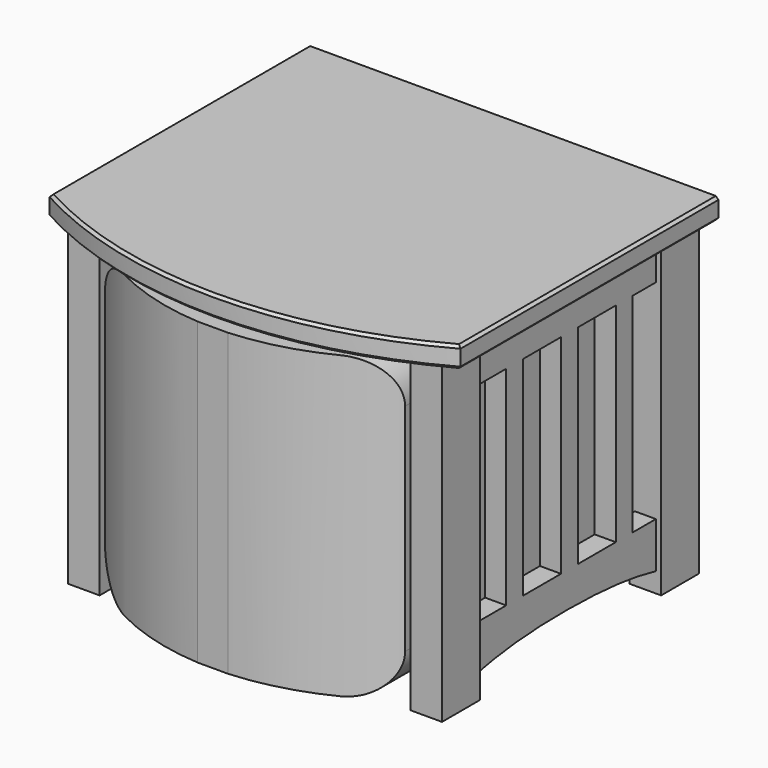
from build123d import *

# Parameters (mm, degrees)
F4_DEPTH  = 425.45
F5_R      = 19.05
F6_DEPTH  = 9.525
F8_DEPTH  = 361.95
F9_W      = 57.15
F9_H      = 381.0128062427
F10_DEPTH = 38.1
F9_H_2    = 381
F11_W     = 57.15
F11_H     = 251.1923307657
F12_DEPTH = 25.4
F16_DEPTH = 25.4
F17_SIZE  = 3.175
F18_W     = 374.65
F18_H     = 25.4
F19_DEPTH = 19.05


# Not quite as in the source:
# - a feature names something its author has since deleted; it is built from what else it names


with BuildPart() as f4:
    # F3 (on Front) → F4 (new body)
    with BuildSketch(Plane.XZ):
        with BuildLine():
            ThreePointArc((0, 50.8), (14.8789755157, 14.8789755157), (50.8, 0))
            Line((50.8, 0), (311.15, 0))
            ThreePointArc((311.15, 0), (347.0710244843, 14.8789755157), (361.95, 50.8))
            Line((361.95, 50.8), (361.95, 311.15))
            ThreePointArc((361.95, 311.15), (347.0710244843, 347.0710244843), (311.15, 361.95))
            Line((311.15, 361.95), (50.8, 361.95))
            ThreePointArc((50.8, 361.95), (14.8789755157, 347.0710244843), (0, 311.15))
            Line((0, 311.15), (0, 50.8))
        make_face()
    extrude(amount=F4_DEPTH)

    # F5 (on face) → F6 (join)
    with BuildSketch(Plane(origin=(0, 0, 0), x_dir=(1, 0, 0), z_dir=(0, 0, -1))):
        with Locations((97.1778258681, 312.0730817318)):
            Circle(F5_R)
        with Locations((274.7920155525, 310.3018701077)):
            Circle(F5_R)
        with Locations((273.9252448082, 45.0676828623)):
            Circle(F5_R)
        with Locations((99.7027978301, 47.6680137217)):
            Circle(F5_R)
    extrude(amount=F6_DEPTH)

    # F7 (on face) → F8 (cut)
    with BuildSketch(Plane.XY.offset(361.95)):
        with BuildLine():
            Line((0, -361.95), (0, -425.45))
            Line((0, -425.45), (0, -444.5584714413))
            Line((0, -444.5584714413), (361.95, -444.5584714413))
            Line((361.95, -444.5584714413), (361.95, -425.45))
            Line((361.95, -425.45), (361.95, -361.95))
            ThreePointArc((361.95, -361.95), (180.975, -426.0410288054), (0, -361.95))
        make_face()
    extrude(amount=-F8_DEPTH, mode=Mode.SUBTRACT)


with BuildPart() as f10:
    # F9 (on offset) → F10 (new body)
    with BuildSketch(Plane.YZ.offset(-6.35)):
        with Locations((-3.175, 180.9685968786)):
            Rectangle(F9_W, F9_H)
    extrude(amount=-F10_DEPTH)



with BuildPart() as f10b:
    # F9 (on offset) → F10, piece 2 (new body)
    with BuildSketch(Plane.YZ.offset(-6.35)):
        with Locations((-333.375, 180.9621937573)):
            Rectangle(F9_W, F9_H_2)
    extrude(amount=-F10_DEPTH)


with BuildPart() as f10_1:
    add(f10.part)

    add(f10b.part)  # F12 merges F10b
    # F11 (on offset) → F12 (join)
    with BuildSketch(Plane.YZ.offset(-12.7)):
        with BuildLine():
            add(Edge.make_bspline(
                [(-31.75, 14.161660336), (-75.4469480959, 24.607324823), (-170.5375424164, 30.3344869468), (-261.7136147626, 24.4613710426), (-304.8, 14.161660336)],
                knots=[0, 0, 0, 0, 0.5035177426, 1, 1, 1, 1], degree=3))
            Line((-31.75, 14.161660336), (-31.75, 69.4826692343))
            Line((-31.75, 69.4826692343), (-66.7540449142, 69.4826692343))
            Line((-66.7540449142, 69.4826692343), (-66.7540449142, 320.675))
            Line((-66.7540449142, 320.675), (-31.75, 320.675))
            Line((-31.75, 320.675), (-31.75, 371.475))
            Line((-31.75, 371.475), (-304.8, 371.475))
            Line((-304.8, 371.475), (-304.8, 371.4621937573))
            Line((-304.8, 371.4621937573), (-304.8, 320.675))
            Line((-304.8, 320.675), (-257.2540449142, 320.675))
            Line((-257.2540449142, 320.675), (-257.2540449142, 69.4826692343))
            Line((-257.2540449142, 69.4826692343), (-304.8, 69.4826692343))
            Line((-304.8, 69.4826692343), (-304.8, 14.161660336))
        make_face()
        with Locations((-203.2790449142, 195.0788346171)):
            Rectangle(F11_W, F11_H, mode=Mode.SUBTRACT)
        with Locations((-120.7290449142, 195.0788346171)):
            Rectangle(F11_W, F11_H, mode=Mode.SUBTRACT)
    extrude(amount=-F12_DEPTH)


with BuildPart() as f13_1:
    # F13: instance of F10
    add(f10_1.part.mirror(Plane.YZ.offset(180.975)))


with BuildPart() as f10_2:
    add(f10_1.part)

    add(f13_1.part)  # F16 merges F13_1
    # F15 (on offset) → F16 (join)
    with BuildSketch(Plane.XY.offset(371.4621937573)):
        with BuildLine():
            Line((-66.675, 26.8077049404), (-66.675, 0))
            Line((-66.675, 0), (-66.675, -361.95))
            ThreePointArc((-66.675, -361.95), (180.975, -425.45), (428.625, -361.95))
            Line((428.625, -361.95), (428.625, 0))
            Line((428.625, 0), (428.625, 26.8077049404))
            Line((428.625, 26.8077049404), (-66.675, 26.8077049404))
        make_face()
    extrude(amount=F16_DEPTH)

    # F17
    f17_edges = [f10_2.edges().sort_by_distance(p)[0] for p in [
        (428.625, -167.571148, 396.862194),
        (180.975, -425.45, 396.862194),
        (-66.675, -167.571148, 396.862194),
        (428.625, -167.571148, 371.462194),
        (180.975, -425.45, 371.462194),
        (-66.675, -167.571148, 371.462194),
    ]]
    chamfer(f17_edges, length=F17_SIZE)

    # F18 (on face) → F19 (join)
    with BuildSketch(Plane(origin=(0, 25.4, 0), x_dir=(-1, 0, 0), z_dir=(0, 1, 0))):
        with Locations((-180.975, 358.7621937573)):
            Rectangle(F18_W, F18_H)
        with Locations((-180.975, 53.9621937573)):
            Rectangle(F18_W, F18_H)
    extrude(amount=-F19_DEPTH)


solid = Compound([f4.part, f10_2.part])
